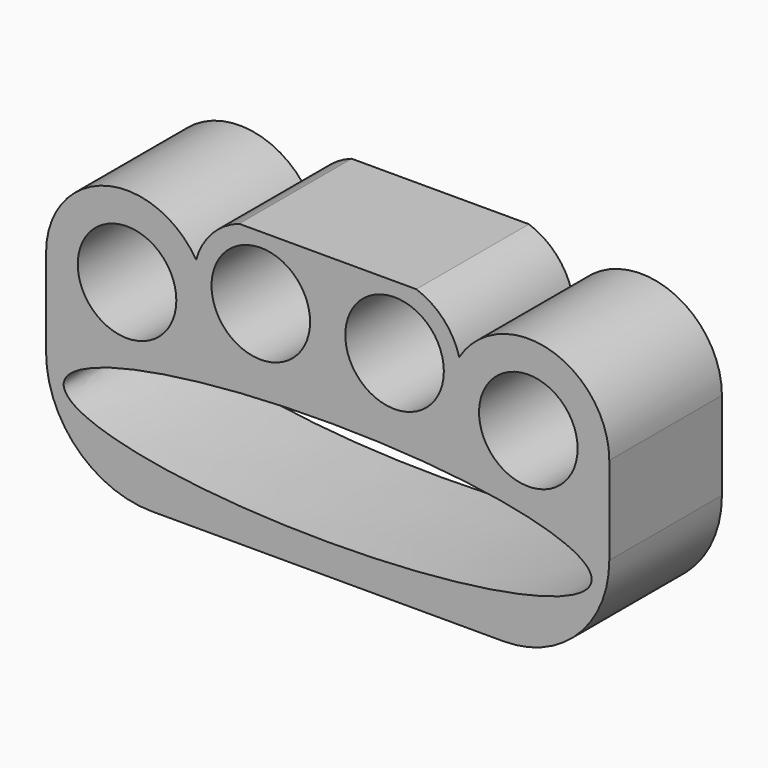
from build123d import *

# Parameters (mm, degrees)
F0_W     = 101.6
F0_H     = 50.8
F0_R     = 8.89
F1_DEPTH = 25.4
F2_R     = 19.05
F4_DEPTH = 25.4


# Not quite as in the source:
# - a feature of the source that left no trace in its solid (it failed there, or was rolled back) is left out


with BuildPart() as f1:
    # F0 (on Front) → F1 (new body)
    with BuildSketch(Plane.XZ):
        Rectangle(F0_W, F0_H)
        with BuildLine():
            add(Edge.make_bspline(
                [(47.625, -10.414), (47.625, 6.0837839421), (-23.8125, -2.165108029), (-95.25, -10.414), (-23.8125, -18.662891971), (47.625, -26.9117839421), (47.625, -10.414)],
                knots=[0, 0, 0, 2.0943951024, 2.0943951024, 4.1887902048, 4.1887902048, 6.2831853072, 6.2831853072, 6.2831853072], degree=2, weights=[1, 0.5, 1, 0.5, 1, 0.5, 1]))
        make_face(mode=Mode.SUBTRACT)
        with Locations((-36.195, 9.525)):
            Circle(F0_R, mode=Mode.SUBTRACT)
        with Locations((-12.065, 13.97)):
            Circle(F0_R, mode=Mode.SUBTRACT)
        with Locations((36.195, 9.525)):
            Circle(F0_R, mode=Mode.SUBTRACT)
        with Locations((12.065, 13.97)):
            Circle(F0_R, mode=Mode.SUBTRACT)
    extrude(amount=F1_DEPTH)

    # F2
    f2_edges = [f1.edges().sort_by_distance(p)[0] for p in [
        (50.8, -12.7, -25.4),
        (-50.8, -12.7, -25.4),
    ]]
    fillet(f2_edges, radius=F2_R)

    # F3 (on face) → F4 (cut)
    with BuildSketch(Plane.XZ.offset(25.4)):
        with BuildLine():
            ThreePointArc((-23.7253094007, 17.1284756105), (-20.880833481, 22.2295316779), (-15.9757395084, 25.4))
            Line((-15.9757395084, 25.4), (-50.8, 25.4))
            Line((-50.8, 25.4), (-50.8, 9.525))
            ThreePointArc((-50.8, 9.525), (-40.1438095547, 23.5860429237), (-23.7253094007, 17.1284756105))
        make_face()
        with BuildLine():
            Line((50.8, 25.4), (15.9757395084, 25.4))
            ThreePointArc((15.9757395084, 25.4), (20.880833481, 22.2295316779), (23.7253094007, 17.1284756105))
            ThreePointArc((23.7253094007, 17.1284756105), (40.1438095547, 23.5860429237), (50.8, 9.525))
            Line((50.8, 9.525), (50.8, 25.4))
        make_face()
    extrude(amount=-F4_DEPTH, mode=Mode.SUBTRACT)


solid = f1.part
